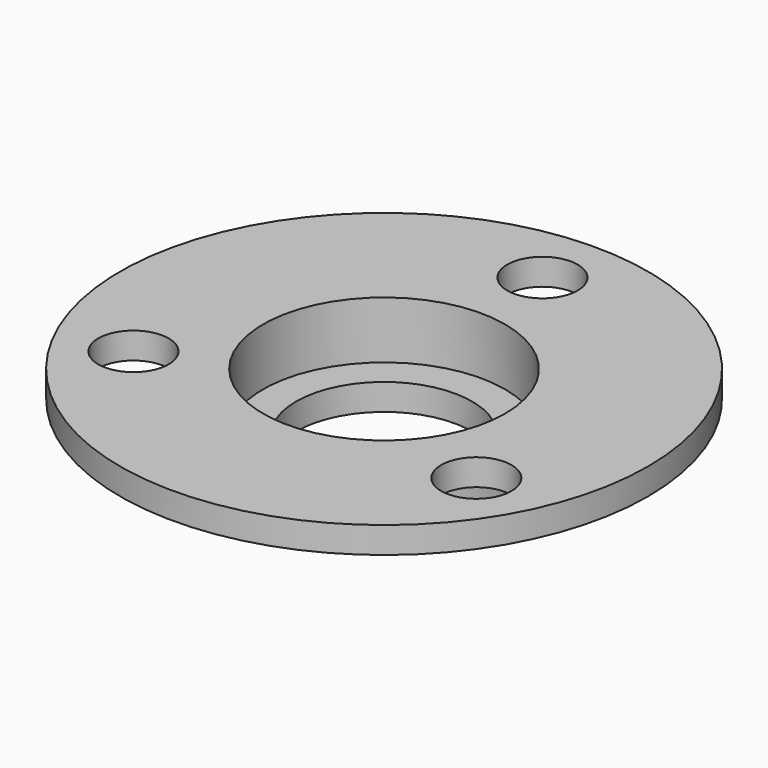
from build123d import *

# Parameters (mm, degrees)
F0_R           = 15.25
F1_DEPTH       = 9.5
F2_R           = 30
F3_DEPTH       = 3
F4_DEPTH       = 3
F5_DEPTH       = 3
F6_D           = 8
F6_DEPTH       = 5
F6_TIP         = 2.4034424761
F7_D           = 8
F7_DEPTH       = 5
F7_TIP         = 2.4034424761
F8_D           = 8
F8_DEPTH       = 5
F8_TIP         = 2.4034424761
F9_D           = 20
F9_DEPTH       = 50
F9_CBORE_D     = 27.5
F9_CBORE_DEPTH = 6.5
F9_TIP         = 6.0086061903


with BuildPart() as f1:
    # F0 (on Top) → F1 (new body)
    with BuildSketch(Plane.XY):
        Circle(F0_R)
    extrude(amount=F1_DEPTH)



with BuildPart() as f3:
    # F2 (on face) → F3 (new body)
    with BuildSketch(Plane.XY.offset(9.5)):
        Circle(F2_R)
        with BuildLine():
            ThreePointArc((0, 22.5), (15.9099025767, 15.9099025767), (22.5, 0))
            ThreePointArc((22.5, 0), (21.7333310915, -5.8234285148), (19.4855715851, -11.25))
            ThreePointArc((19.4855715851, -11.25), (0, -22.5), (-19.4855715851, -11.25))
            ThreePointArc((-19.4855715851, -11.25), (-19.4855715851, 11.25), (0, 22.5))
        make_face(mode=Mode.SUBTRACT)
    extrude(amount=-F3_DEPTH)


with BuildPart() as f1_1:
    add(f1.part)

    add(f3.part)  # F3#2 merges F3
    # F2 (on face) → F3, piece 2 (join)
    with BuildSketch(Plane.XY.offset(9.5)):
        with BuildLine():
            Line((-14.8906008631, -3.2912772501), (-19.4855715851, -11.25))
            Line((-19.4855715851, -11.25), (-10.295630141, -11.25))
            ThreePointArc((-10.295630141, -11.25), (-13.2068874077, -7.625), (-14.8906008631, -3.2912772501))
        make_face()
    extrude(amount=-F3_DEPTH)

    # F2 (on face) → F4 (join)
    with BuildSketch(Plane.XY.offset(9.5)):
        with BuildLine():
            Line((-4.5949707221, 14.5412772501), (0, 22.5))
            ThreePointArc((0, 22.5), (-19.4855715851, 11.25), (-19.4855715851, -11.25))
            Line((-19.4855715851, -11.25), (-14.8906008631, -3.2912772501))
            ThreePointArc((-14.8906008631, -3.2912772501), (-13.2068874077, 7.625), (-4.5949707221, 14.5412772501))
        make_face()
        with BuildLine():
            ThreePointArc((-19.4855715851, -11.25), (0, -22.5), (19.4855715851, -11.25))
            Line((19.4855715851, -11.25), (10.295630141, -11.25))
            ThreePointArc((10.295630141, -11.25), (0, -15.25), (-10.295630141, -11.25))
            Line((-10.295630141, -11.25), (-19.4855715851, -11.25))
        make_face()
        with BuildLine():
            ThreePointArc((19.4855715851, -11.25), (21.7333310915, -5.8234285148), (22.5, 0))
            ThreePointArc((22.5, 0), (15.9099025767, 15.9099025767), (0, 22.5))
            Line((0, 22.5), (4.5949707221, 14.5412772501))
            ThreePointArc((4.5949707221, 14.5412772501), (12.3011341654, 9.0135785482), (15.25, 0))
            ThreePointArc((15.25, 0), (15.1598839567, -1.655420919), (14.8906008631, -3.2912772501))
            Line((14.8906008631, -3.2912772501), (19.4855715851, -11.25))
        make_face()
    extrude(amount=-F4_DEPTH)

    # F2 (on face) → F5 (join)
    with BuildSketch(Plane.XY.offset(9.5)):
        with BuildLine():
            Line((4.5949707221, 14.5412772501), (0, 22.5))
            Line((0, 22.5), (-4.5949707221, 14.5412772501))
            ThreePointArc((-4.5949707221, 14.5412772501), (0, 15.25), (4.5949707221, 14.5412772501))
        make_face()
        with BuildLine():
            ThreePointArc((-19.4855715851, -11.25), (0, -22.5), (19.4855715851, -11.25))
            Line((19.4855715851, -11.25), (10.295630141, -11.25))
            ThreePointArc((10.295630141, -11.25), (0, -15.25), (-10.295630141, -11.25))
            Line((-10.295630141, -11.25), (-19.4855715851, -11.25))
        make_face()
        with BuildLine():
            Line((10.295630141, -11.25), (19.4855715851, -11.25))
            Line((19.4855715851, -11.25), (14.8906008631, -3.2912772501))
            ThreePointArc((14.8906008631, -3.2912772501), (13.2068874077, -7.625), (10.295630141, -11.25))
        make_face()
    extrude(amount=-F5_DEPTH)

    # F6
    with Locations(Plane.XY.offset(9.5)):
        with Locations((-19.4855715851, -11.25)):
            Hole(F6_D / 2, depth=F6_DEPTH)
            with Locations((0, 0, -(F6_DEPTH + F6_TIP / 2))):  # 118° drill point
                Cone(0, F6_D / 2, F6_TIP, mode=Mode.SUBTRACT)

    # F7
    with Locations(Plane.XY.offset(9.5)):
        with Locations((0, 22.5)):
            Hole(F7_D / 2, depth=F7_DEPTH)
            with Locations((0, 0, -(F7_DEPTH + F7_TIP / 2))):  # 118° drill point
                Cone(0, F7_D / 2, F7_TIP, mode=Mode.SUBTRACT)

    # F8
    with Locations(Plane.XY.offset(9.5)):
        with Locations((19.4855715851, -11.25)):
            Hole(F8_D / 2, depth=F8_DEPTH)
            with Locations((0, 0, -(F8_DEPTH + F8_TIP / 2))):  # 118° drill point
                Cone(0, F8_D / 2, F8_TIP, mode=Mode.SUBTRACT)

    # F9
    with Locations(Plane.XY.offset(9.5)):
        with Locations((0, 0)):
            CounterBoreHole(F9_D / 2, F9_CBORE_D / 2, F9_CBORE_DEPTH, depth=F9_DEPTH)
            with Locations((0, 0, -(F9_DEPTH + F9_TIP / 2))):  # 118° drill point
                Cone(0, F9_D / 2, F9_TIP, mode=Mode.SUBTRACT)


solid = f1_1.part
